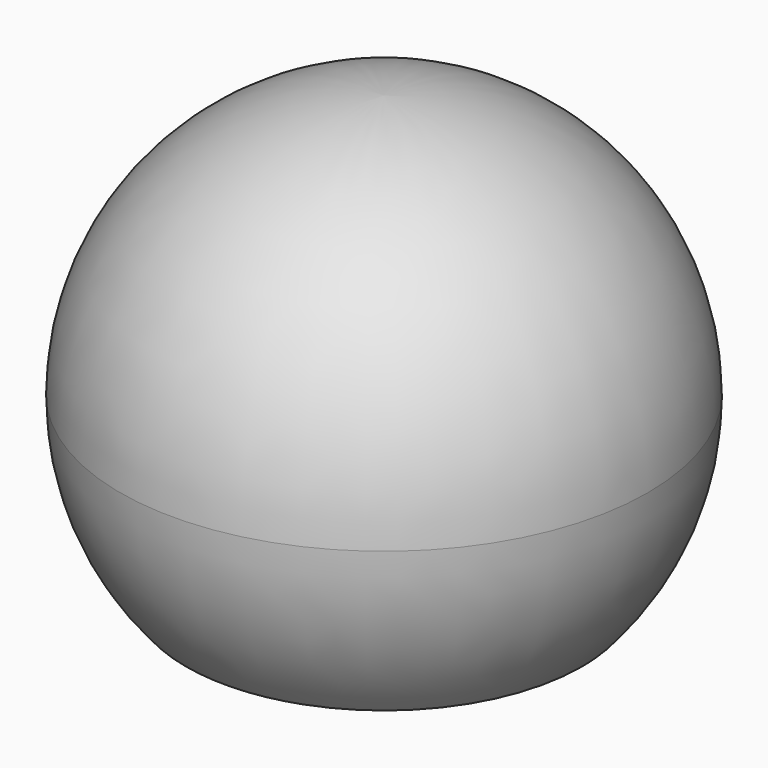
from build123d import *

# Parameters (mm, degrees)
F0_R     = 10
F1_DEPTH = 20
F2_R     = 9.99999
F3_R     = 7.5
F4_DEPTH = 10.39


# Not quite as in the source:
# - a fillet or chamfer is up to 0.001 mm smaller than in the source, because OpenCascade refuses the exact size


with BuildPart() as f1:
    # F0 (on Top) → F1 (new body)
    with BuildSketch(Plane.XY):
        Circle(F0_R)
    extrude(amount=F1_DEPTH)

    # F2 (radius 10 in the source; OpenCascade refuses exactly that, so slightly less here)
    f2_edges = [f1.edges().sort_by_distance(p)[0] for p in [
        (-10, 0, 20),
        (-10, 0, 0),
    ]]
    fillet(f2_edges, radius=F2_R)

    # F3 (on Top) → F4 (cut)
    with BuildSketch(Plane.XY):
        Circle(F3_R)
    extrude(amount=F4_DEPTH, mode=Mode.SUBTRACT)


solid = f1.part
